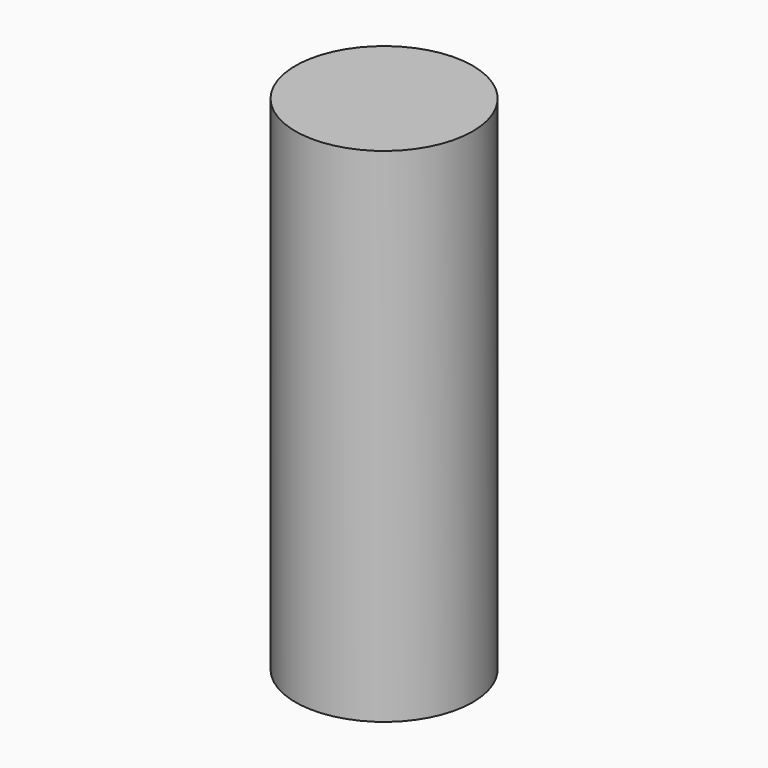
from build123d import *

# Parameters (mm, degrees)
F0_W         = 30
F0_H         = 30
F1_DEPTH     = 30
F3_DEPTH     = 15
F4_T1_DEPTH  = 39
F4_T3_DEPTH  = 39
F4_T5_DEPTH  = 18
F4_S9_W      = 6.12
F4_S9_H      = 6.12
F4_T10_DEPTH = 6.12
F4_S15_W     = 6.12
F4_S15_H     = 6.12
F4_T16_DEPTH = 6.12
F5_TEXT_SIZE = 12.2384701912
F6_DEPTH     = 2
F7_W         = 55.6632075459
F7_H         = 51.417702809
F8_DEPTH     = 50
F11_R        = 30
F12_DEPTH    = 170


# Not quite as in the source:
# - a fillet or chamfer that OpenCascade refuses, or shapes differently, is made with other operations: its cross-section is extruded or revolved along the edge and cut away or added
# - a feature of the source that left no trace in its solid (it failed there, or was rolled back) is left out
# - Text() gives the source's letters only with a copy of the font that has no kerning and outlines rounded to 1/6400 em; it was checked with that copy


with BuildPart() as f1:
    # F0 (on Top) → F1 (new body)
    with BuildSketch(Plane.XY):
        with Locations((-15, 15)):
            Rectangle(F0_W, F0_H)
    extrude(amount=F1_DEPTH)

    # F2 (on face) → F3 (cut)
    with BuildSketch(Plane(origin=(-30, 0, 0), x_dir=(0, -1, 0), z_dir=(-1, 0, 0))):
        with BuildLine():
            ThreePointArc((-22.0710678119, 7.9289321881), (-15, 5), (-7.9289321881, 7.9289321881))
            Line((-7.9289321881, 7.9289321881), (-15, 15))
            Line((-15, 15), (-22.0710678119, 7.9289321881))
        make_face()
        with BuildLine():
            Line((-15, 15), (-7.9289321881, 7.9289321881))
            ThreePointArc((-7.9289321881, 7.9289321881), (-5.7612046749, 11.1731656763), (-5, 15))
            ThreePointArc((-5, 15), (-5.7612046749, 18.8268343237), (-7.9289321881, 22.0710678119))
            Line((-7.9289321881, 22.0710678119), (-15, 15))
        make_face()
        with BuildLine():
            Line((-22.0710678119, 7.9289321881), (-15, 15))
            Line((-15, 15), (-22.0710678119, 22.0710678119))
            ThreePointArc((-22.0710678119, 22.0710678119), (-25, 15), (-22.0710678119, 7.9289321881))
        make_face()
        with BuildLine():
            Line((-22.0710678119, 22.0710678119), (-15, 15))
            Line((-15, 15), (-7.9289321881, 22.0710678119))
            ThreePointArc((-7.9289321881, 22.0710678119), (-15, 25), (-22.0710678119, 22.0710678119))
        make_face()
    extrude(amount=-F3_DEPTH, mode=Mode.SUBTRACT)

    # F4: fillet of radius 6 on 6 edges, made by hand

    # F4_s2 → F4_t1 (cut)
    with BuildSketch(Plane.YZ.offset(-24)):
        with BuildLine():
            ThreePointArc((24, 30), (28.2426406871, 28.2426406871), (30, 24))
            Line((30, 24), (30, 30))
            Line((30, 30), (24, 30))
        make_face()
        with BuildLine():
            ThreePointArc((24, 0), (28.2426406871, 1.7573593129), (30, 6))
            Line((30, 6), (30, 0))
            Line((30, 0), (24, 0))
        make_face()
    extrude(amount=F4_T1_DEPTH, mode=Mode.SUBTRACT)

    # F4_s4 → F4_t3 (cut)
    with BuildSketch(Plane.XZ.offset(-24)):
        with BuildLine():
            ThreePointArc((-30, 6), (-28.2426406871, 1.7573593129), (-24, 0))
            Line((-24, 0), (-30, 0))
            Line((-30, 0), (-30, 6))
        make_face()
        with BuildLine():
            ThreePointArc((-30, 24), (-28.2426406871, 28.2426406871), (-24, 30))
            Line((-24, 30), (-30, 30))
            Line((-30, 30), (-30, 24))
        make_face()
    extrude(amount=F4_T3_DEPTH, mode=Mode.SUBTRACT)

    # F4_s6 → F4_t5 (cut)
    with BuildSketch(Plane.XY.offset(6)):
        with BuildLine():
            ThreePointArc((-30, 24), (-28.2426406871, 28.2426406871), (-24, 30))
            Line((-24, 30), (-30, 30))
            Line((-30, 30), (-30, 24))
        make_face()
    extrude(amount=F4_T5_DEPTH, mode=Mode.SUBTRACT)


with BuildPart() as f4_tool8:
    # F4_s9 → F4_t10 (new body)
    with BuildSketch(Plane.YZ.offset(-24)):
        with Locations((27.06, 27.06)):
            Rectangle(F4_S9_W, F4_S9_H)
    extrude(amount=-F4_T10_DEPTH)

    # F4_s11 → F4_t12 (revolve, cut)
    with BuildSketch(Plane(origin=(-24, 24, 24), x_dir=(0, -0.7071067812, -0.7071067812), z_dir=(0, 0.7071067812, -0.7071067812))):
        with BuildLine():
            ThreePointArc((0, -6), (6, 0), (0, 6))
            Line((0, 6), (0, -6))
        make_face()
    revolve(axis=Axis((-24, 24, 24), (-1, 0, 0)), mode=Mode.SUBTRACT)


with BuildPart() as f1_1:
    add(f1.part)

    # F4_t7: cut F4_tool8
    add(f4_tool8.part, mode=Mode.SUBTRACT)


with BuildPart() as f4_tool14:
    # F4_s15 → F4_t16 (new body)
    with BuildSketch(Plane.YZ.offset(-24)):
        with Locations((27.06, 2.94)):
            Rectangle(F4_S15_W, F4_S15_H)
    extrude(amount=-F4_T16_DEPTH)

    # F4_s17 → F4_t18 (revolve, cut)
    with BuildSketch(Plane(origin=(-24, 24, 6), x_dir=(0, -0.7071067812, 0.7071067812), z_dir=(0, -0.7071067812, -0.7071067812))):
        with BuildLine():
            ThreePointArc((0, -6), (6, 0), (0, 6))
            Line((0, 6), (0, -6))
        make_face()
    revolve(axis=Axis((-24, 24, 6), (-1, 0, 0)), mode=Mode.SUBTRACT)


with BuildPart() as f1_2:
    add(f1_1.part)

    # F4_t13: cut F4_tool14
    add(f4_tool14.part, mode=Mode.SUBTRACT)

    # F5 (on face) → F6 (join)
    with BuildSketch(Plane.XZ):
        with Locations((-22.9068806395, 10.6458705481)):
            Text('DV', F5_TEXT_SIZE, font='Open Sans', text_align=(TextAlign.LEFT, TextAlign.BOTTOM))
    extrude(amount=F6_DEPTH)

    # F7 (on Right) → F8 (join)
    with BuildSketch(Plane.YZ):
        with Locations((16.7056573555, 15.1579631492)):
            Rectangle(F7_W, F7_H)
    extrude(amount=-F8_DEPTH)


with BuildPart() as f12:
    # F11 (on Top) → F12 (new body)
    with BuildSketch(Plane.XY):
        Circle(F11_R)
    extrude(amount=F12_DEPTH)


solid = f12.part
